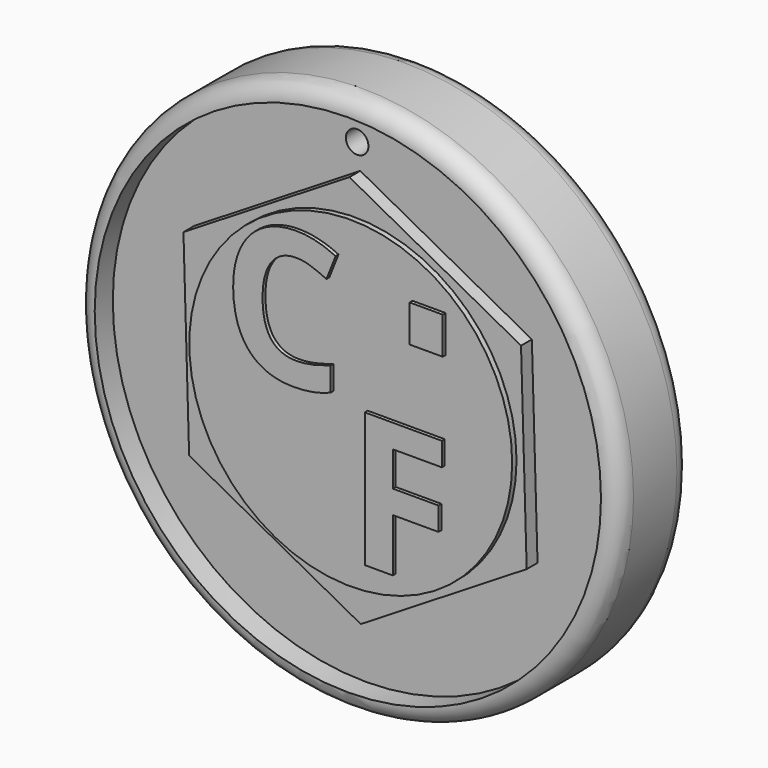
from build123d import *

# Parameters (mm, degrees)
F0_R         = 76.2
F1_DEPTH     = 25.4
F2_R         = 5.08
F3_DEPTH     = 6.35
F4_TEXT_SIZE = 52.9166666667
F6_DEPTH     = 6.35
F5_TEXT_SIZE = 52.9166666667
F7_DEPTH     = 6.35
F9_R         = 3.175
F10_DEPTH    = 25.4
F12_DEPTH    = 3.81
F14_W        = 9.3096345663
F14_H        = 10.4134455323
F15_DEPTH    = 2.54
F19_R        = 45.3628352666
F20_DEPTH    = 1.524


# Not quite as in the source:
# - the program builds the solid bodies; features that only make, move or delete a surface that nothing else refers to are left out
# - Text() gives the source's letters only with a copy of the font that has no kerning and outlines rounded to 1/6400 em; it was checked with that copy


with BuildPart() as f1:
    # F0 (on Front) → F1 (new body)
    with BuildSketch(Plane.XZ):
        Circle(F0_R)
    extrude(amount=F1_DEPTH)

    # F2
    f2_edges = [f1.edges().sort_by_distance(p)[0] for p in [
        (-76.2, -25.4, 0),
        (-76.2, 0, 0),
    ]]
    fillet(f2_edges, radius=F2_R)

    # F3 (cut): a face of the model
    f3_faces = [f1.faces().sort_by_distance(p)[0] for p in [
        (0, -25.4, 0),
    ]]
    extrude(f3_faces, amount=-F3_DEPTH, mode=Mode.SUBTRACT)

    # F4 (on face) → F6 (join)
    with BuildSketch(Plane.XZ.offset(19.05)):
        with Locations((-35.2888020833, 0)):
            Text('C', F4_TEXT_SIZE, font='Open Sans', font_style=FontStyle.BOLD, text_align=(TextAlign.LEFT, TextAlign.BOTTOM))
    extrude(amount=F6_DEPTH)

    # F5 (on face) → F7 (join)
    with BuildSketch(Plane.XZ.offset(19.05)):
        with Locations((0, -38.1)):
            Text('F', F5_TEXT_SIZE, font='Open Sans', font_style=FontStyle.BOLD, text_align=(TextAlign.LEFT, TextAlign.BOTTOM))
    extrude(amount=F7_DEPTH)

    # F9 (on face) → F10 (cut)
    with BuildSketch(Plane.XZ.offset(19.05)):
        with Locations((-2.4622979108, 61.6217963398)):
            Circle(F9_R)
    extrude(amount=-F10_DEPTH, mode=Mode.SUBTRACT)

    # F11 (on face) → F12 (join)
    with BuildSketch(Plane.XZ.offset(19.05)):
        Polygon((46.6230730341, 28.753957403), (-1.5901210533, 54.7537443516), (-48.2131940874, 25.9997869485), (-46.6230730341, -28.753957403), (1.5901210533, -54.7537443516), (48.2131940874, -25.9997869485), align=None)
    extrude(amount=F12_DEPTH)

    # F14 (on face) → F15 (join)
    with BuildSketch(Plane.XZ.offset(22.86)):
        with Locations((22.0039300621, 25.7518924773)):
            Rectangle(F14_W, F14_H)
    extrude(amount=F15_DEPTH)

    # F19 (on face) → F20 (join)
    with BuildSketch(Plane.XZ.offset(22.86)):
        Circle(F19_R)
    extrude(amount=F20_DEPTH)


solid = f1.part
